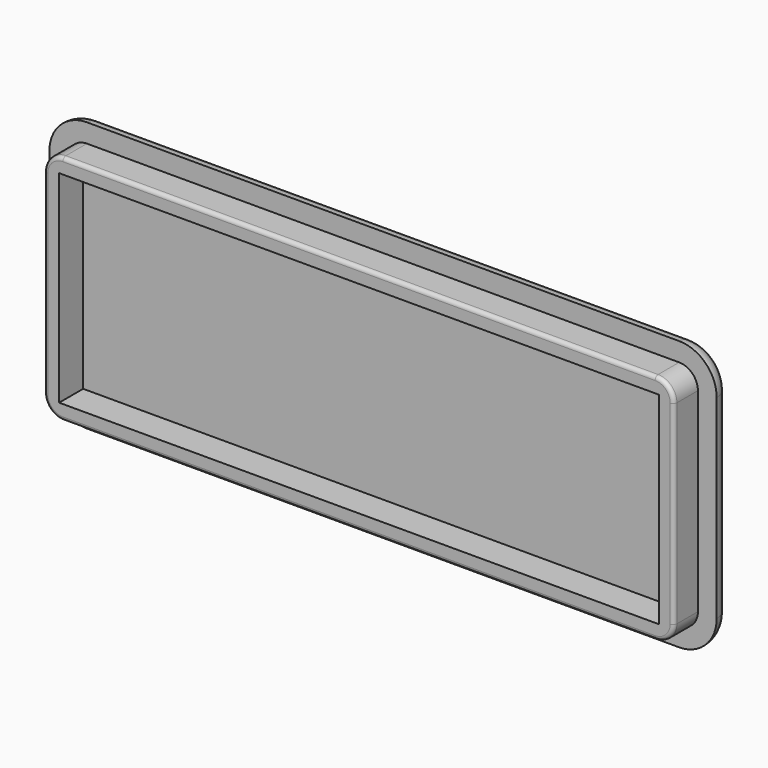
from build123d import *

# Parameters (mm, degrees)
F2_W     = 88.9
F2_H     = 35.9210244843
F3_DEPTH = 2.5
F4_R     = 5
F5_W     = 83.9
F5_H     = 30.9210244843
F5_W_2   = 79.9
F5_H_2   = 26.9210244843
F6_DEPTH = 4
F7_R     = 2.5
F8_R     = 2.49999
F9_R     = 0.5


# Not quite as in the source:
# - a fillet or chamfer is up to 0.001 mm smaller than in the source, because OpenCascade refuses the exact size


with BuildPart() as f3:
    # F2 (on Front) → F3 (new body)
    with BuildSketch(Plane.XZ):
        Rectangle(F2_W, F2_H)
    extrude(amount=-F3_DEPTH)

    # F4
    f4_edges = [f3.edges().sort_by_distance(p)[0] for p in [
        (44.45, 1.25, 17.960512),
        (44.45, 1.25, -17.960512),
        (-44.45, 1.25, -17.960512),
        (-44.45, 1.25, 17.960512),
    ]]
    fillet(f4_edges, radius=F4_R)

    # F5 (on Front) → F6 (join)
    with BuildSketch(Plane.XZ):
        Rectangle(F5_W, F5_H)
        Rectangle(F5_W_2, F5_H_2, mode=Mode.SUBTRACT)
    extrude(amount=F6_DEPTH)

    # F7
    f7_edges = [f3.edges().sort_by_distance(p)[0] for p in [
        (-41.95, -2, -15.460512),
        (-41.95, -2, 15.460512),
        (41.95, -2, -15.460512),
        (41.95, -2, 15.460512),
    ]]
    fillet(f7_edges, radius=F7_R)

    # F8 (radius 2.5 in the source; OpenCascade refuses exactly that, so slightly less here)
    f8_edges = [f3.edges().sort_by_distance(p)[0] for p in [
        (0, 2.5, -17.960512),
    ]]
    fillet(f8_edges, radius=F8_R)

    # F9
    f9_edges = [f3.edges().sort_by_distance(p)[0] for p in [
        (41.95, -4, 0),
    ]]
    fillet(f9_edges, radius=F9_R)


solid = f3.part
